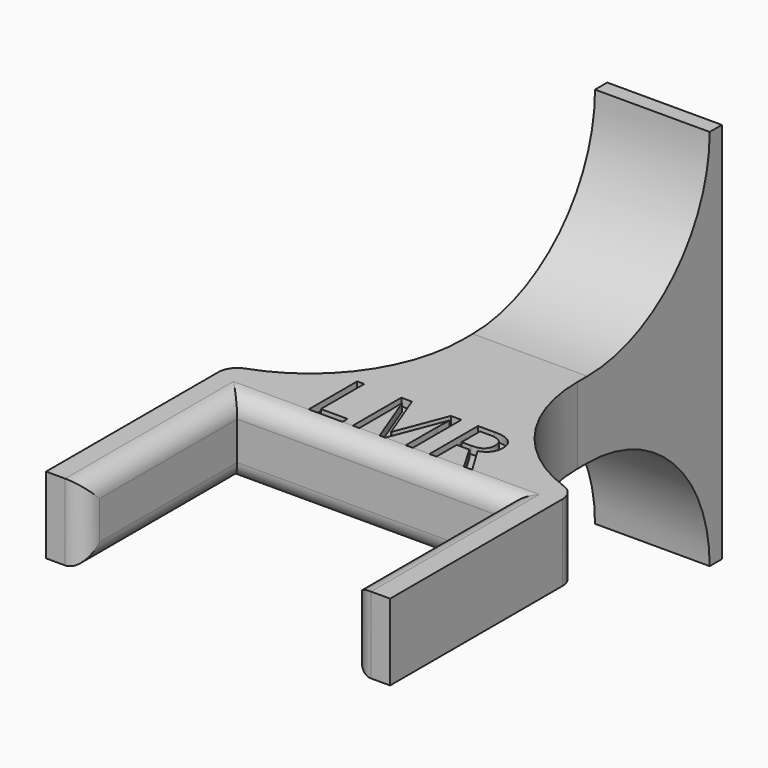
from build123d import *

# Parameters (mm, degrees)
F0_W         = 15
F0_H         = 41
F0_W_2       = 5
F0_H_2       = 25
F1_DEPTH     = 5
F0_H_3       = 2
F2_DEPTH     = 25
F3_T1_DEPTH  = 15
F3_T3_DEPTH  = 10
F4_R         = 2.5
F5_TEXT_SIZE = 11.1111111111
F6_DEPTH     = 1


# Not quite as in the source:
# - a fillet or chamfer that OpenCascade refuses, or shapes differently, is made with other operations: its cross-section is extruded or revolved along the edge and cut away or added
# - Text() gives the source's letters only with a copy of the font that has no kerning and outlines rounded to 1/6400 em; it was checked with that copy


with BuildPart() as f1:
    # F0 (on Top) → F1 (new body, symmetric)
    with BuildSketch(Plane.XY):
        with Locations((0, 38)):
            Rectangle(F0_W, F0_H)
        Polygon((-22.5, 12.5), (-17.5, 12.5), (17.5, 12.5), (22.5, 12.5), (22.5, 17.5), (7.5, 17.5), (-7.5, 17.5), (-22.5, 17.5), align=None)
        with Locations((20, 0)):
            Rectangle(F0_W_2, F0_H_2)
        with Locations((-20, 0)):
            Rectangle(F0_W_2, F0_H_2)
    extrude(amount=F1_DEPTH, both=True)

    # F0 (on Top) → F2 (join, symmetric)
    with BuildSketch(Plane.XY):
        with Locations((0, 59.5)):
            Rectangle(F0_W, F0_H_3)
    extrude(amount=F2_DEPTH, both=True)

    # F3: fillet of radius 20 on 4 edges, made by hand

    # F3_s2 → F3_t1 (join)
    with BuildSketch(Plane.YZ.offset(-7.5)):
        with BuildLine():
            ThreePointArc((58.5, 25), (52.6421356237, 10.8578643763), (38.5, 5))
            Line((38.5, 5), (58.5, 5))
            Line((58.5, 5), (58.5, 25))
        make_face()
        with BuildLine():
            ThreePointArc((58.5, -25), (52.6421356237, -10.8578643763), (38.5, -5))
            Line((38.5, -5), (58.5, -5))
            Line((58.5, -5), (58.5, -25))
        make_face()
    extrude(amount=F3_T1_DEPTH)

    # F3_s4 → F3_t3 (join)
    with BuildSketch(Plane.XY.offset(-5)):
        with BuildLine():
            ThreePointArc((7.5, 36.864916731), (11.6886116992, 24.6174680171), (22.5, 17.5))
            Line((22.5, 17.5), (7.5, 17.5))
            Line((7.5, 17.5), (7.5, 36.864916731))
        make_face()
        with BuildLine():
            ThreePointArc((-7.5, 36.864916731), (-11.6886116992, 24.6174680171), (-22.5, 17.5))
            Line((-22.5, 17.5), (-7.5, 17.5))
            Line((-7.5, 17.5), (-7.5, 36.864916731))
        make_face()
    extrude(amount=F3_T3_DEPTH)

    # F4
    f4_edges = [f1.edges().sort_by_distance(p)[0] for p in [
        (17.5, -12.5, 0),
        (-17.5, -12.5, 0),
        (22.5, 17.5, 0),
        (-22.5, 17.5, 0),
        (-17.5, 0, -5),
        (-17.5, 0, 5),
        (17.5, 0, -5),
        (17.5, 0, 5),
        (0, 12.5, 5),
        (0, 12.5, -5),
    ]]
    fillet(f4_edges, radius=F4_R)

    # F5 (on face) → F6 (cut)
    with BuildSketch(Plane.XY.offset(5)):
        with Locations((-11.2387152778, 15)):
            Text('LMR', F5_TEXT_SIZE, font='Open Sans', text_align=(TextAlign.LEFT, TextAlign.BOTTOM))
    extrude(amount=-F6_DEPTH, mode=Mode.SUBTRACT)


solid = f1.part
